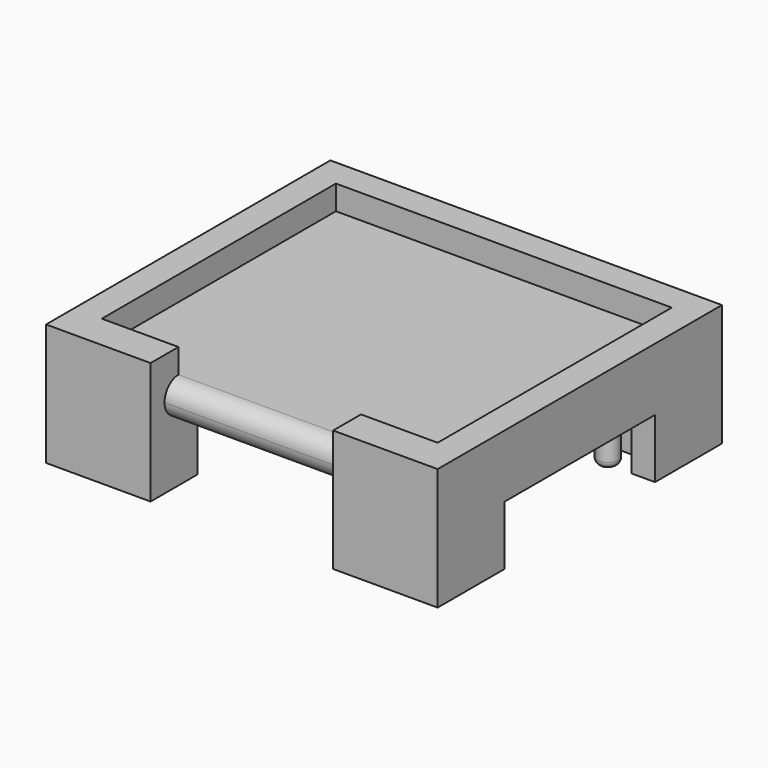
from build123d import *

# Parameters (mm, degrees)
F0_W     = 26.2
F0_H     = 2.5
F1_DEPTH = 5
F2_DEPTH = 8.5
F4_DEPTH = 9
F3_R     = 1.5
F5_DEPTH = 9
F6_R     = 1
F7_R     = 2.49999


# Not quite as in the source:
# - a fillet or chamfer is up to 0.001 mm smaller than in the source, because OpenCascade refuses the exact size


with BuildPart() as f1:
    # F0 (on Top) → F1 (new body)
    with BuildSketch(Plane.XY):
        Polygon((13.1, -20.5), (23.1, -20.5), (24.1, -20.5), (24.1, 21.5), (-24.1, 21.5), (-24.1, -20.5), (-23.1, -20.5), (-13.1, -20.5), align=None)
        with Locations((0, -21.75)):
            Rectangle(F0_W, F0_H)
        Polygon((-13.1, -23), (-13.1, -20.5), (-23.1, -20.5), (-24.1, -20.5), (-28.1, -20.5), (-28.1, -25.5), (-13.1, -25.5), align=None)
    extrude(amount=F1_DEPTH)

    # F0 (on Top) → F2 (join)
    with BuildSketch(Plane.XY):
        Polygon((24.1, -20.5), (23.1, -20.5), (13.1, -20.5), (13.1, -23), (13.1, -25.5), (28.1, -25.5), (28.1, -20.5), align=None)
        Polygon((24.1, 21.5), (24.1, -20.5), (28.1, -20.5), (28.1, 25.5), (-28.1, 25.5), (-28.1, -20.5), (-24.1, -20.5), (-24.1, 21.5), align=None)
        Polygon((-13.1, -23), (-13.1, -20.5), (-23.1, -20.5), (-24.1, -20.5), (-28.1, -20.5), (-28.1, -25.5), (-13.1, -25.5), align=None)
    extrude(amount=F2_DEPTH)

    # F3 (on face) → F4 (join)
    with BuildSketch(Plane(origin=(0, 0, 0), x_dir=(1, 0, 0), z_dir=(0, 0, -1))):
        Polygon((-28.1, 13.5), (-24.75, 13.5), (-24.75, 17.1), (-13.1, 17.1), (-13.1, 23), (-13.1, 25.5), (-28.1, 25.5), align=None)
        Polygon((-19.0010517836, -25.5), (-19.0010517836, -17.1), (-24.75, -17.1), (-24.75, -13.5), (-28.1, -13.5), (-28.1, -25.5), align=None)
        Polygon((24.75, -13.5), (24.75, -17.1), (16.1, -17.1), (16.1, -25.5), (28.1, -25.5), (28.1, -13.5), align=None)
        Polygon((24.75, 17.1), (24.75, 13.5), (28.1, 13.5), (28.1, 25.5), (13.1, 25.5), (13.1, 23), (13.1, 17.1), align=None)
    extrude(amount=F4_DEPTH)

    # F3 (on face) + F2_face1 (on face) → F5 (join)
    with BuildSketch(Plane(origin=(0, 0, 0), x_dir=(1, 0, 0), z_dir=(0, 0, -1))):
        with Locations((-21.25, 13.6)):
            Circle(F3_R)
        with Locations((-21.25, -13.6)):
            Circle(F3_R)
        with Locations((21.25, -13.6)):
            Circle(F3_R)
        with Locations((21.25, 13.6)):
            Circle(F3_R)
    with BuildSketch(Plane(origin=(0, 2.8148564997, 8.5), x_dir=(1, 0, 0), z_dir=(0, 0, 1))):
        Polygon((24.1, -23.3148564997), (13.1, -23.3148564997), (13.1, -28.3148564997), (28.1, -28.3148564997), (28.1, 22.6851435003), (-28.1, 22.6851435003), (-28.1, -28.3148564997), (-13.1, -28.3148564997), (-13.1, -23.3148564997), (-24.1, -23.3148564997), (-24.1, 18.6851435003), (24.1, 18.6851435003), align=None)
    extrude(amount=F5_DEPTH, dir=(0, 0, -1))

    # F6
    f6_edges = [f1.edges().sort_by_distance(p)[0] for p in [
        (-22.75, 13.6, -9),
        (-22.75, -13.6, -9),
        (19.75, -13.6, -9),
        (19.75, 13.6, -9),
    ]]
    fillet(f6_edges, radius=F6_R)

    # F7 (radius 2.5 in the source; OpenCascade refuses exactly that, so slightly less here)
    f7_edges = [f1.edges().sort_by_distance(p)[0] for p in [
        (0, -23, 0),
        (0, -23, 5),
    ]]
    fillet(f7_edges, radius=F7_R)


solid = f1.part
